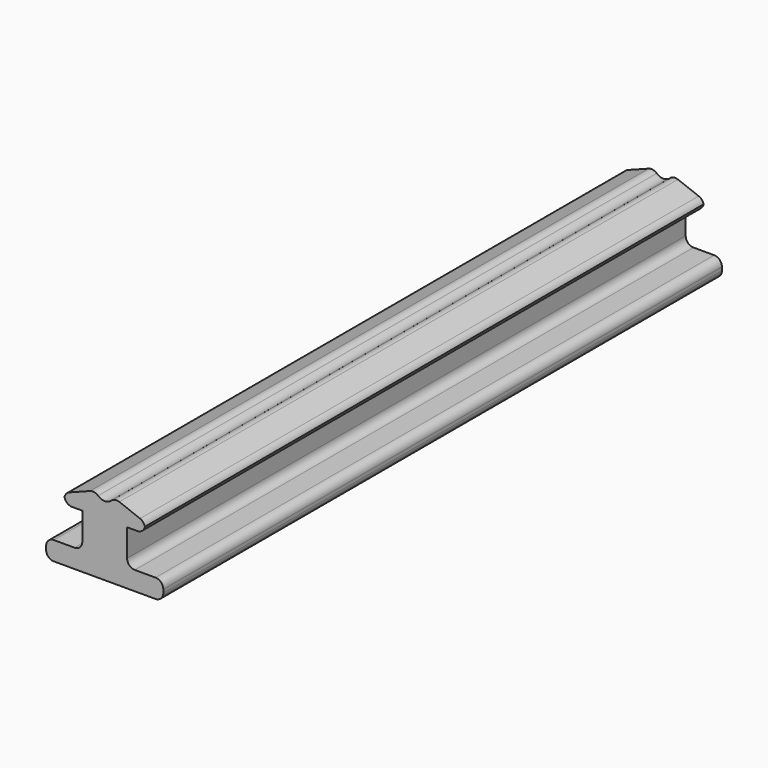
from build123d import *

# Parameters (mm, degrees)
F1_DEPTH    = 227.8918027878
F3_D        = 12.7
F4_T1_DEPTH = 455.7836055756
F4_T3_DEPTH = 473.2454690546
F4_T5_DEPTH = 481.1836055756
F4_T7_DEPTH = 475.2289422773


# Not quite as in the source:
# - a fillet or chamfer that OpenCascade refuses, or shapes differently, is made with other operations: its cross-section is extruded or revolved along the edge and cut away or added


with BuildPart() as f1:
    # F0 (on Front) → F1 (new body, symmetric)
    with BuildSketch(Plane.XZ):
        Polygon((-38.2542312145, 0), (0, 0), (38.2542312145, 0), (38.2542312145, 12.2701972723), (14.6159976721, 12.2701972723), (14.6159976721, 35.1866483688), (26.3448953629, 35.1866483688), (26.3448953629, 41.6826456785), (0, 51.7875403166), (-26.3448953629, 41.6826456785), (-26.3448953629, 35.1866483688), (-14.6159976721, 35.1866483688), (-14.6159976721, 12.2701972723), (-38.2542312145, 12.2701972723), align=None)
    extrude(amount=F1_DEPTH, both=True)

    # F3 (through all)
    with Locations(Plane.XZ.offset(227.8918027878)):
        with Locations((0, 51.7875403166)):
            Hole(F3_D / 2)

    # F4: fillet of radius 5.08 on 12 edges, made by hand

    # F4_s2 → F4_t1 (join)
    with BuildSketch(Plane.XZ.offset(-227.8918027878)):
        with BuildLine():
            ThreePointArc((-19.6959976721, 12.2701972723), (-16.1038952237, 13.7580948239), (-14.6159976721, 17.3501972723))
            Line((-14.6159976721, 17.3501972723), (-14.6159976721, 12.2701972723))
            Line((-14.6159976721, 12.2701972723), (-19.6959976721, 12.2701972723))
        make_face()
        with BuildLine():
            ThreePointArc((14.6159976721, 17.3501972723), (16.1038952237, 13.7580948239), (19.6959976721, 12.2701972723))
            Line((19.6959976721, 12.2701972723), (14.6159976721, 12.2701972723))
            Line((14.6159976721, 12.2701972723), (14.6159976721, 17.3501972723))
        make_face()
    extrude(amount=F4_T1_DEPTH)

    # F4_s4 → F4_t3 (cut)
    with BuildSketch(Plane.XZ.offset(-236.6227345273)):
        with BuildLine():
            ThreePointArc((23.0841549326, 42.9333410423), (25.4510773115, 41.0681681672), (26.3448953629, 38.1902729827))
            Line((26.3448953629, 38.1902729827), (26.3448953629, 41.6826456785))
            Line((26.3448953629, 41.6826456785), (23.0841549326, 42.9333410423))
        make_face()
        with BuildLine():
            ThreePointArc((-26.3448953629, 38.1902729827), (-25.4510773115, 41.0681681672), (-23.0841549326, 42.9333410423))
            Line((-23.0841549326, 42.9333410423), (-26.3448953629, 41.6826456785))
            Line((-26.3448953629, 41.6826456785), (-26.3448953629, 38.1902729827))
        make_face()
    extrude(amount=F4_T3_DEPTH, mode=Mode.SUBTRACT)

    # F4_s6 → F4_t5 (cut)
    with BuildSketch(Plane.XZ.offset(-240.5918027878)):
        with BuildLine():
            ThreePointArc((26.3448953629, 40.2666483688), (24.8569978113, 36.6745459204), (21.2648953629, 35.1866483688))
            Line((21.2648953629, 35.1866483688), (26.3448953629, 35.1866483688))
            Line((26.3448953629, 35.1866483688), (26.3448953629, 40.2666483688))
        make_face()
        with BuildLine():
            ThreePointArc((-21.2648953629, 35.1866483688), (-24.8569978113, 36.6745459204), (-26.3448953629, 40.2666483688))
            Line((-26.3448953629, 40.2666483688), (-26.3448953629, 35.1866483688))
            Line((-26.3448953629, 35.1866483688), (-21.2648953629, 35.1866483688))
        make_face()
        with BuildLine():
            ThreePointArc((38.2542312145, 7.1901972723), (36.766333663, 10.7822997207), (33.1742312145, 12.2701972723))
            Line((33.1742312145, 12.2701972723), (38.2542312145, 12.2701972723))
            Line((38.2542312145, 12.2701972723), (38.2542312145, 7.1901972723))
        make_face()
        with BuildLine():
            ThreePointArc((33.1742312145, 0), (36.766333663, 1.4878975516), (38.2542312145, 5.08))
            Line((38.2542312145, 5.08), (38.2542312145, 0))
            Line((38.2542312145, 0), (33.1742312145, 0))
        make_face()
        with BuildLine():
            ThreePointArc((-38.2542312145, 7.1901972723), (-36.766333663, 10.7822997207), (-33.1742312145, 12.2701972723))
            Line((-33.1742312145, 12.2701972723), (-38.2542312145, 12.2701972723))
            Line((-38.2542312145, 12.2701972723), (-38.2542312145, 7.1901972723))
        make_face()
        with BuildLine():
            ThreePointArc((-33.1742312145, 0), (-36.766333663, 1.4878975516), (-38.2542312145, 5.08))
            Line((-38.2542312145, 5.08), (-38.2542312145, 0))
            Line((-38.2542312145, 0), (-33.1742312145, 0))
        make_face()
    extrude(amount=F4_T5_DEPTH, mode=Mode.SUBTRACT)

    # F4_s8 → F4_t7 (cut)
    with BuildSketch(Plane.XZ.offset(-237.6144711386)):
        with BuildLine():
            ThreePointArc((-9.5599593035, 48.120705426), (-6.7869567139, 48.367304114), (-4.300388741, 47.1153720109))
            ThreePointArc((-4.300388741, 47.1153720109), (-5.2532816874, 48.2202540213), (-5.9288350745, 49.5134658544))
            Line((-5.9288350745, 49.5134658544), (-9.5599593035, 48.120705426))
        make_face()
        with BuildLine():
            ThreePointArc((4.300388741, 47.1153720109), (6.7869567139, 48.367304114), (9.5599593035, 48.120705426))
            Line((9.5599593035, 48.120705426), (5.9288350745, 49.5134658544))
            ThreePointArc((5.9288350745, 49.5134658544), (5.2532816874, 48.2202540213), (4.300388741, 47.1153720109))
        make_face()
    extrude(amount=F4_T7_DEPTH, mode=Mode.SUBTRACT)


solid = f1.part
